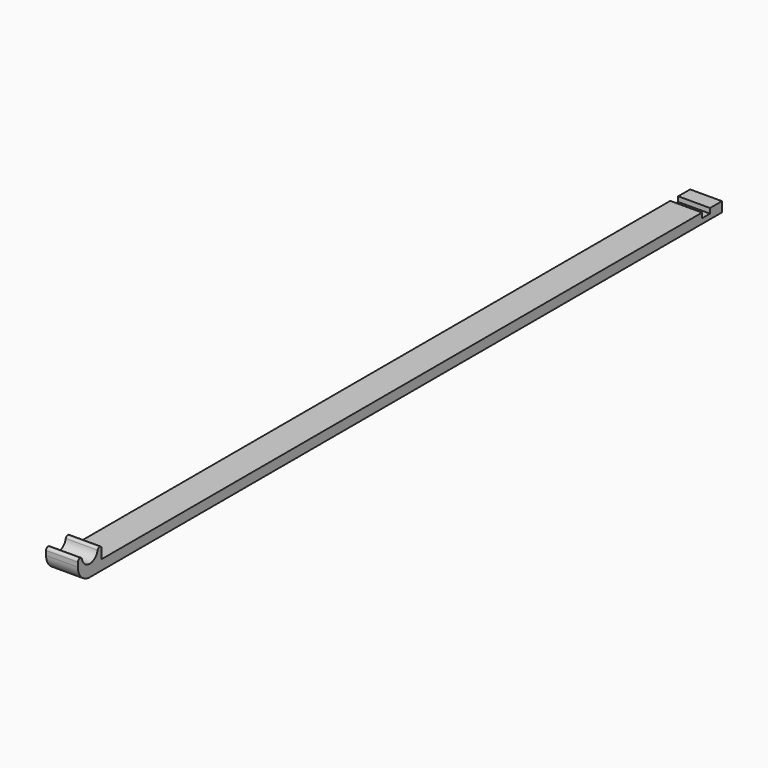
from build123d import *

# Parameters (mm, degrees)
F1_DEPTH = 6.4


# Not quite as in the source:
# - a feature names something its author has since deleted; it is built from what else it names


with BuildPart() as f1:
    # F0 (on Right) → F1 (new body)
    with BuildSketch(Plane.YZ):
        with BuildLine():
            Line((-159, 0), (0, 0))
            Line((0, 0), (0, 2))
            Line((0, 2), (-3, 2))
            Line((-3, 2), (-3, 1))
            Line((-3, 1), (-5, 1))
            Line((-5, 1), (-5, 2))
            Line((-5, 2), (-156, 2))
            Line((-156, 2), (-156, 3.9))
            ThreePointArc((-156, 3.9), (-156.1464466094, 4.2535533906), (-156.5, 4.4))
            Line((-156.5, 4.4), (-156.5505102572, 4.4))
            ThreePointArc((-156.5505102572, 4.4), (-156.8667380232, 4.2872983346), (-157.0404082058, 4))
            ThreePointArc((-157.0404082058, 4), (-159, 2.4), (-160.9595917942, 4))
            ThreePointArc((-160.9595917942, 4), (-161.1332619768, 4.2872983346), (-161.4494897428, 4.4))
            Line((-161.4494897428, 4.4), (-161.5, 4.4))
            ThreePointArc((-161.5, 4.4), (-161.8535533906, 4.2535533906), (-162, 3.9))
            Line((-162, 3.9), (-162, 3))
            ThreePointArc((-162, 3), (-161.1213203436, 0.8786796564), (-159, 0))
        make_face()
    extrude(amount=F1_DEPTH)


solid = f1.part
